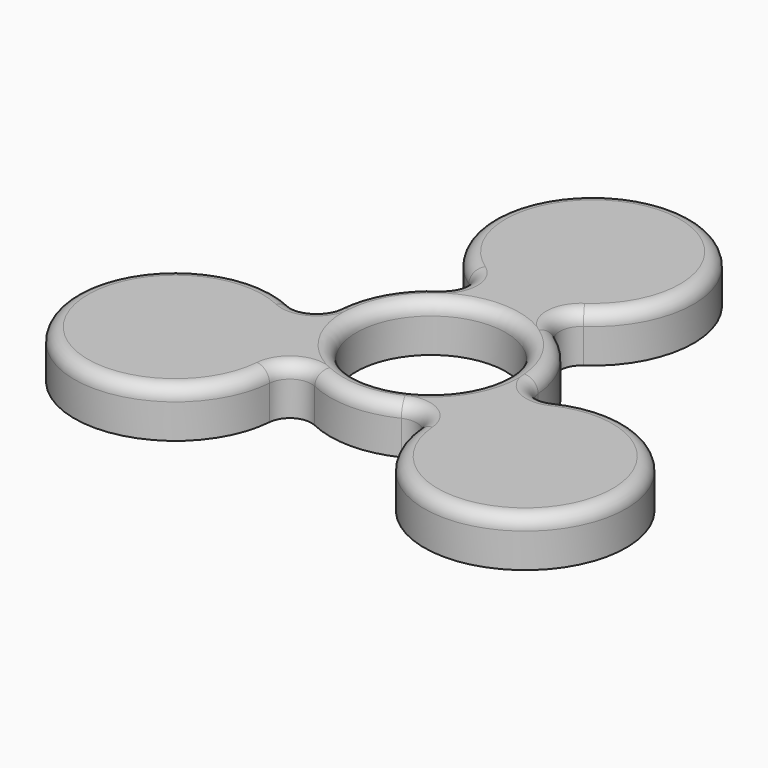
from build123d import *

# Parameters (mm, degrees)
F0_R         = 15
F0_R_2       = 11.1125
F1_DEPTH     = 7.1
F2_R         = 15
F3_DEPTH     = 7.1
F5_DEPTH     = 7.1
F6_T2_ANGLE  = 50.822828172
F6_T4_ANGLE  = 110.822828172
F6_T6_ANGLE  = 290.822828172
F6_T8_ANGLE  = 110.822828172
F6_T10_ANGLE = 50.822828172
F6_T12_ANGLE = 110.822828172
F6_T14_ANGLE = 290.822828172
F6_T16_ANGLE = 110.822828172
F6_T18_ANGLE = 50.822828172
F6_T20_ANGLE = 110.822828172
F6_T22_ANGLE = 290.822828172
F6_T24_ANGLE = 110.822828172


# Not quite as in the source:
# - a fillet or chamfer that OpenCascade refuses, or shapes differently, is made with other operations: its cross-section is extruded or revolved along the edge and cut away or added


with BuildPart() as f1:
    # F0 (on Top) → F1 (new body)
    with BuildSketch(Plane.XY):
        Circle(F0_R)
        Circle(F0_R_2, mode=Mode.SUBTRACT)
    extrude(amount=F1_DEPTH)

    # F2 (on Top) → F3 (join)
    with BuildSketch(Plane.XY):
        with Locations((0, 30)):
            Circle(F2_R)
        with Locations((-25.9807621135, -15)):
            Circle(F2_R)
        with Locations((25.9807621135, -15)):
            Circle(F2_R)
    extrude(amount=F3_DEPTH)

    # F4 (on Top) → F5 (join)
    with BuildSketch(Plane.XY):
        with BuildLine():
            ThreePointArc((8.5151963101, 17.6512578859), (4.459196579, 15.6781437701), (-3.4e-09, 15))
            ThreePointArc((-3.4e-09, 15), (4.459196579, 14.3218562299), (8.5151963101, 12.3487421141))
            ThreePointArc((8.5151963101, 12.3487421141), (7.1229179094, 15), (8.5151963101, 17.6512578859))
        make_face()
        with BuildLine():
            ThreePointArc((-8.5151963101, 17.6512578859), (-7.1229179094, 15), (-8.5151963101, 12.3487421141))
            ThreePointArc((-8.5151963101, 12.3487421141), (-4.4591965822, 14.3218562289), (-3.4e-09, 15))
            ThreePointArc((-3.4e-09, 15), (-4.4591965822, 15.6781437711), (-8.5151963101, 17.6512578859))
        make_face()
        with BuildLine():
            ThreePointArc((-12.9903811554, -7.4999998292), (-14.632689636, -3.2991504992), (-14.9519225306, 1.2000052657))
            ThreePointArc((-14.9519225306, 1.2000052657), (-16.5518400115, -1.3313721414), (-19.544035893, -1.4512526202))
            ThreePointArc((-19.544035893, -1.4512526202), (-15.8072691523, -3.9772942992), (-12.9903811554, -7.4999998292))
        make_face()
        with BuildLine():
            ThreePointArc((-6.4367262205, -13.5487473798), (-10.1734931062, -11.0227055671), (-12.9903811554, -7.4999998292))
            ThreePointArc((-12.9903811554, -7.4999998292), (-11.3480725209, -11.7008493083), (-11.0288395829, -16.2000052657))
            ThreePointArc((-11.0288395829, -16.2000052657), (-9.4289221021, -13.6686278586), (-6.4367262205, -13.5487473798))
        make_face()
        with BuildLine():
            ThreePointArc((12.9903809901, -7.5000001155), (10.1734929847, -11.0227056792), (6.4367262205, -13.5487473798))
            ThreePointArc((6.4367262205, -13.5487473798), (9.4289221021, -13.6686278586), (11.0288395829, -16.2000052657))
            ThreePointArc((11.0288395829, -16.2000052657), (11.3480724846, -11.7008494696), (12.9903809901, -7.5000001155))
        make_face()
        with BuildLine():
            ThreePointArc((14.9519225306, 1.2000052657), (14.6326895996, -3.2991506605), (12.9903809901, -7.5000001155))
            ThreePointArc((12.9903809901, -7.5000001155), (15.8072690308, -3.9772944113), (19.544035893, -1.4512526202))
            ThreePointArc((19.544035893, -1.4512526202), (16.5518400115, -1.3313721414), (14.9519225306, 1.2000052657))
        make_face()
    extrude(amount=F5_DEPTH)

    # F6: fillet of radius 2 on 13 edges, made by hand

    # F6_s1 → F6_t2 (revolve, cut)
    with BuildSketch(Plane(origin=(0, 0, 0), x_dir=(0, 0, 1), z_dir=(-0.8232494743, 0.567679754, 0))):
        with BuildLine():
            ThreePointArc((5.1, 15), (6.5142135624, 14.4142135624), (7.1, 13))
            Line((7.1, 13), (7.1, 15))
            Line((7.1, 15), (5.1, 15))
        make_face()
    revolve(axis=Axis((0, 0, 7.1), (0, 0, -1)), revolution_arc=F6_T2_ANGLE, mode=Mode.SUBTRACT)

    # F6_s3 → F6_t4 (revolve, cut)
    with BuildSketch(Plane(origin=(0, 0, 0), x_dir=(0, 0, 1), z_dir=(0.8232494743, -0.567679754, 0))):
        with BuildLine():
            ThreePointArc((7.1, -13), (6.5142135624, -14.4142135624), (5.1, -15))
            Line((5.1, -15), (7.1, -15))
            Line((7.1, -15), (7.1, -13))
        make_face()
    revolve(axis=Axis((10.3433972036, 15, 7.1), (0, 0, -1)), revolution_arc=F6_T4_ANGLE, mode=Mode.SUBTRACT)

    # F6_s5 → F6_t6 (revolve, cut)
    with BuildSketch(Plane(origin=(14.0202617712, 9.6678090933, 0), x_dir=(0, 0, 1), z_dir=(-0.8232494743, -0.567679754, 0))):
        with BuildLine():
            ThreePointArc((5.1, 9.6974842282), (6.5142135624, 10.2832706658), (7.1, 11.6974842282))
            Line((7.1, 11.6974842282), (7.1, 9.6974842282))
            Line((7.1, 9.6974842282), (5.1, 9.6974842282))
        make_face()
    revolve(axis=Axis((0, 30, 7.1), (0, 0, 1)), revolution_arc=F6_T6_ANGLE, mode=Mode.SUBTRACT)

    # F6_s7 → F6_t8 (revolve, cut)
    with BuildSketch(Plane(origin=(-14.0202617712, 9.6678090933, 0), x_dir=(0, 0, 1), z_dir=(-0.8232494743, 0.567679754, 0))):
        with BuildLine():
            ThreePointArc((5.1, 9.6974842282), (6.5142135624, 10.2832706658), (7.1, 11.6974842282))
            Line((7.1, 11.6974842282), (7.1, 9.6974842282))
            Line((7.1, 9.6974842282), (5.1, 9.6974842282))
        make_face()
    revolve(axis=Axis((-10.3433972036, 15, 7.1), (0, 0, -1)), revolution_arc=F6_T8_ANGLE, mode=Mode.SUBTRACT)

    # F6_s9 → F6_t10 (revolve, cut)
    with BuildSketch(Plane(origin=(0, 0, 0), x_dir=(0, 0, 1), z_dir=(0.8232494743, 0.567679754, 0))):
        with BuildLine():
            ThreePointArc((5.1, -15), (6.5142135624, -14.4142135624), (7.1, -13))
            Line((7.1, -13), (7.1, -15))
            Line((7.1, -15), (5.1, -15))
        make_face()
    revolve(axis=Axis((0, 0, 7.1), (0, 0, 1)), revolution_arc=F6_T10_ANGLE, mode=Mode.SUBTRACT)

    # F6_s11 → F6_t12 (revolve, cut)
    with BuildSketch(Plane(origin=(0, 0, 0), x_dir=(0, 0, 1), z_dir=(0.080000351, 0.9967948354, 0))):
        with BuildLine():
            ThreePointArc((5.1, -15), (6.5142135624, -14.4142135624), (7.1, -13))
            Line((7.1, -13), (7.1, -15))
            Line((7.1, -15), (5.1, -15))
        make_face()
    revolve(axis=Axis((-18.1620796586, 1.4576447398, 7.1), (0, 0, -1)), revolution_arc=F6_T12_ANGLE, mode=Mode.SUBTRACT)

    # F6_s13 → F6_t14 (revolve, cut)
    with BuildSketch(Plane(origin=(-15.3826991593, 7.307998315, 0), x_dir=(0, 0, 1), z_dir=(0.9032498253, -0.4291150814, 0))):
        with BuildLine():
            ThreePointArc((5.1, 9.6974842282), (6.5142135624, 10.2832706658), (7.1, 11.6974842282))
            Line((7.1, 11.6974842282), (7.1, 9.6974842282))
            Line((7.1, 9.6974842282), (5.1, 9.6974842282))
        make_face()
    revolve(axis=Axis((-25.9807621135, -15, 7.1), (0, 0, 1)), revolution_arc=F6_T14_ANGLE, mode=Mode.SUBTRACT)

    # F6_s15 → F6_t16 (revolve, cut)
    with BuildSketch(Plane(origin=(-1.3624373881, -16.9758074082, 0), x_dir=(0, 0, 1), z_dir=(-0.080000351, -0.9967948354, 0))):
        with BuildLine():
            ThreePointArc((5.1, 9.6974842282), (6.5142135624, 10.2832706658), (7.1, 11.6974842282))
            Line((7.1, 11.6974842282), (7.1, 9.6974842282))
            Line((7.1, 9.6974842282), (5.1, 9.6974842282))
        make_face()
    revolve(axis=Axis((-7.8186824549, -16.4576447398, 7.1), (0, 0, -1)), revolution_arc=F6_T16_ANGLE, mode=Mode.SUBTRACT)

    # F6_s17 → F6_t18 (revolve, cut)
    with BuildSketch(Plane(origin=(0, 0, 0), x_dir=(0, 0, 1), z_dir=(-0.9032498253, 0.4291150814, 0))):
        with BuildLine():
            ThreePointArc((5.1, -15), (6.5142135624, -14.4142135624), (7.1, -13))
            Line((7.1, -13), (7.1, -15))
            Line((7.1, -15), (5.1, -15))
        make_face()
    revolve(axis=Axis((0, 0, 7.1), (0, 0, 1)), revolution_arc=F6_T18_ANGLE, mode=Mode.SUBTRACT)

    # F6_s19 → F6_t20 (revolve, cut)
    with BuildSketch(Plane(origin=(0, 0, 0), x_dir=(0, 0, 1), z_dir=(-0.9032498253, -0.4291150814, 0))):
        with BuildLine():
            ThreePointArc((5.1, -15), (6.5142135624, -14.4142135624), (7.1, -13))
            Line((7.1, -13), (7.1, -15))
            Line((7.1, -15), (5.1, -15))
        make_face()
    revolve(axis=Axis((7.8186824549, -16.4576447398, 7.1), (0, 0, -1)), revolution_arc=F6_T20_ANGLE, mode=Mode.SUBTRACT)

    # F6_s21 → F6_t22 (revolve, cut)
    with BuildSketch(Plane(origin=(1.3624373881, -16.9758074082, 0), x_dir=(0, 0, 1), z_dir=(-0.080000351, 0.9967948354, 0))):
        with BuildLine():
            ThreePointArc((5.1, 9.6974842282), (6.5142135624, 10.2832706658), (7.1, 11.6974842282))
            Line((7.1, 11.6974842282), (7.1, 9.6974842282))
            Line((7.1, 9.6974842282), (5.1, 9.6974842282))
        make_face()
    revolve(axis=Axis((25.9807621135, -15, 7.1), (0, 0, 1)), revolution_arc=F6_T22_ANGLE, mode=Mode.SUBTRACT)

    # F6_s23 → F6_t24 (revolve, cut)
    with BuildSketch(Plane(origin=(15.3826991593, 7.307998315, 0), x_dir=(0, 0, 1), z_dir=(0.9032498253, 0.4291150814, 0))):
        with BuildLine():
            ThreePointArc((5.1, 9.6974842282), (6.5142135624, 10.2832706658), (7.1, 11.6974842282))
            Line((7.1, 11.6974842282), (7.1, 9.6974842282))
            Line((7.1, 9.6974842282), (5.1, 9.6974842282))
        make_face()
    revolve(axis=Axis((18.1620796586, 1.4576447398, 7.1), (0, 0, -1)), revolution_arc=F6_T24_ANGLE, mode=Mode.SUBTRACT)

    # F6_s25 → F6_t26 (revolve, cut)
    with BuildSketch(Plane.XZ):
        with BuildLine():
            ThreePointArc((13.1125, 7.1), (11.6982864376, 6.5142135624), (11.1125, 5.1))
            Line((11.1125, 5.1), (11.1125, 7.1))
            Line((11.1125, 7.1), (13.1125, 7.1))
        make_face()
    revolve(axis=Axis((0, 0, 7.1), (0, 0, 1)), mode=Mode.SUBTRACT)


solid = f1.part
